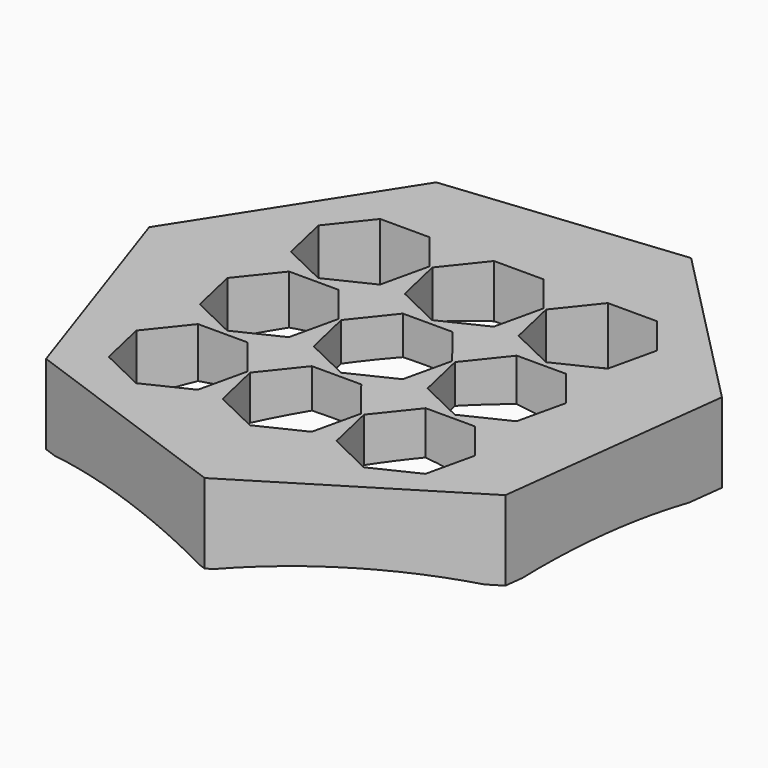
from build123d import *

# Parameters (mm, degrees)
F1_DEPTH = 35


# Not quite as in the source:
# - a feature names something its author has since deleted; it is built from what else it names


with BuildPart() as f1:
    # F0 (on Top) → F1 (new body)
    with BuildSketch(Plane.XY):
        Polygon((113.4119661336, 42.3527422411), (40.5729530569, 116.5079710024), (-62.8183212091, 105.7951663142), (-118.9061183443, 18.2812886083), (-85.4551831235, -80.1339272451), (12.3452479574, -115.3418164038), (100.8494555292, -60.8301202213), align=None)
        Polygon((-74.3810191607, -44.4351838884), (-60.8505664327, -27.4685328169), (-39.1494051825, -27.4685328169), (-25.6189524545, -44.4351838884), (-30.4479151238, -65.592251718), (-49.9999858076, -75.0080327045), (-69.5520564914, -65.592251718), align=None, mode=Mode.SUBTRACT)
        Polygon((-74.3810191607, 5.5648161116), (-60.8505664327, 22.5314671831), (-39.1494051825, 22.5314671831), (-25.6189524545, 5.5648161116), (-30.4479151238, -15.592251718), (-49.9999858076, -25.0080327045), (-69.5520564914, -15.592251718), align=None, mode=Mode.SUBTRACT)
        Polygon((-24.3810191607, -44.4351838884), (-10.8505664327, -27.4685328169), (10.8505948175, -27.4685328169), (24.3810475455, -44.4351838884), (19.5520848762, -65.592251718), (1.41924e-05, -75.0080327045), (-19.5520564914, -65.592251718), align=None, mode=Mode.SUBTRACT)
        Polygon((25.6189808393, -44.4351838884), (39.1494335673, -27.4685328169), (60.8505948175, -27.4685328169), (74.3810475455, -44.4351838884), (69.5520848762, -65.592251718), (50.0000141924, -75.0080327045), (30.4479435086, -65.592251718), align=None, mode=Mode.SUBTRACT)
        Polygon((-24.3810191607, 5.5648161116), (-10.8505664327, 22.5314671831), (10.8505948175, 22.5314671831), (24.3810475455, 5.5648161116), (19.5520848762, -15.592251718), (1.41924e-05, -25.0080327045), (-19.5520564914, -15.592251718), align=None, mode=Mode.SUBTRACT)
        Polygon((25.6189808393, 5.5648161116), (39.1494335673, 22.5314671831), (60.8505948175, 22.5314671831), (74.3810475455, 5.5648161116), (69.5520848762, -15.592251718), (50.0000141924, -25.0080327045), (30.4479435086, -15.592251718), align=None, mode=Mode.SUBTRACT)
        Polygon((-74.3810191607, 55.5648161116), (-60.8505664327, 72.5314671831), (-39.1494051825, 72.5314671831), (-25.6189524545, 55.5648161116), (-30.4479151238, 34.407748282), (-49.9999858076, 24.9919672955), (-69.5520564914, 34.407748282), align=None, mode=Mode.SUBTRACT)
        Polygon((-24.3810191607, 55.5648161116), (-10.8505664327, 72.5314671831), (10.8505948175, 72.5314671831), (24.3810475455, 55.5648161116), (19.5520848762, 34.407748282), (1.41924e-05, 24.9919672955), (-19.5520564914, 34.407748282), align=None, mode=Mode.SUBTRACT)
        Polygon((25.6189808393, 55.5648161116), (39.1494335673, 72.5314671831), (60.8505948175, 72.5314671831), (74.3810475455, 55.5648161116), (69.5520848762, 34.407748282), (50.0000141924, 24.9919672955), (30.4479435086, 34.407748282), align=None, mode=Mode.SUBTRACT)
    extrude(amount=F1_DEPTH)

    # F2 (on Right) → F4 (revolve, cut)
    with BuildSketch(Plane.YZ):
        with BuildLine():
            Line((0, -0.4654330397), (0, 18.9489760594))
            add(Edge.make_bspline(
                [(0, 18.9489760594), (-64.1887508142, 18.9489760594), (-115.3471469879, -0.2508653365)],
                knots=[4.7123889804, 4.7123889804, 4.7123889804, 5.3608745392, 5.3608745392, 5.3608745392], degree=2, weights=[1, 0.9478922419, 1]))
            Line((-115.3471469879, -0.2508653365), (0, -0.4654330397))
        make_face()
    revolve(axis=Axis((0, 0, -8.051071316), (0, 0, -1)), mode=Mode.SUBTRACT)


solid = f1.part
